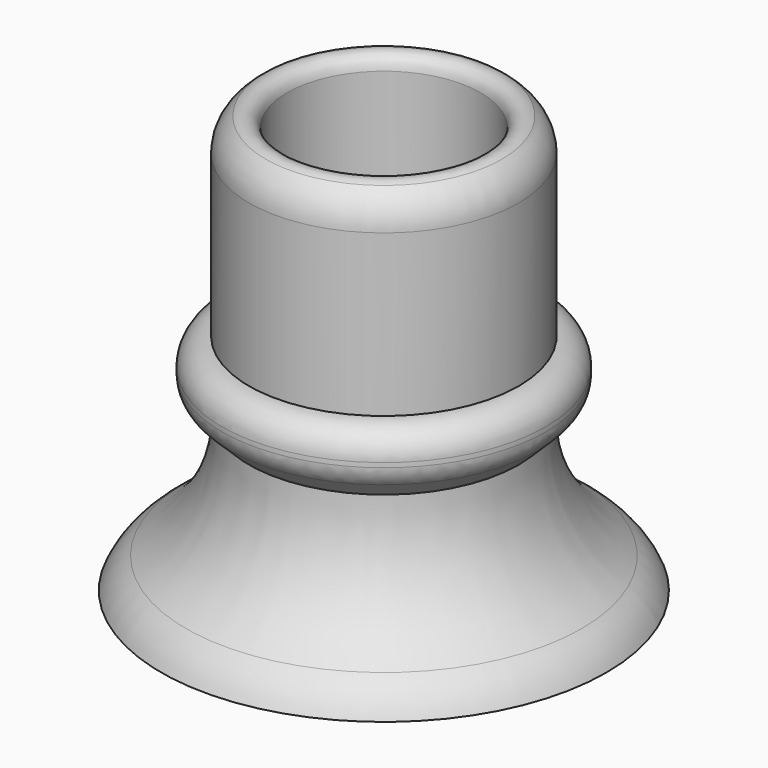
from build123d import *

# Parameters (mm, degrees)
F3_R = 2
F4_R = 2
F6_R = 1


# Not quite as in the source:
# - a fillet or chamfer that OpenCascade refuses, or shapes differently, is made with other operations: its cross-section is extruded or revolved along the edge and cut away or added


with BuildPart() as f1:
    # F0 (on Front) → F1 (revolve)
    with BuildSketch(Plane.XZ):
        with BuildLine():
            ThreePointArc((16.5, 1.2755964417), (11.6628201448, 5.344639677), (10, 11.4430370868))
            Line((10, 11.4430370868), (12, 13.4055894333))
            Line((12, 13.4055894333), (12, 16.5758651609))
            Line((12, 16.5758651609), (9.9997436628, 16.5758651609))
            Line((9.9997436628, 16.5758651609), (9.9997436628, 31.5143950284))
            Line((9.9997436628, 31.5143950284), (7.1613686159, 31.5143950284))
            Line((7.1613686159, 31.5143950284), (7.1613686159, 5.6914240122))
            ThreePointArc((7.1613686159, 5.6914240122), (4.4508587391, 2.967008827), (1, 1.2755964417))
            Line((1, 1.2755964417), (1, 0.0454979338))
            Line((1, 0.0454979338), (16.5, 0))
            Line((16.5, 0), (16.5, 1.2755964417))
        make_face()
    revolve(axis=Axis((0, 0, 19.1986504942), (0, 0, 1)))

    # F2: fillet of radius 5 on 1 edges, made by hand

    # F2_s1 → F2_t2 (revolve, cut)
    with BuildSketch(Plane.XZ):
        with BuildLine():
            ThreePointArc((16.5, 0), (15.750789479, 1.2709297875), (14.6632904097, 2.2678875116))
            ThreePointArc((14.6632904097, 2.2678875116), (15.557168946, 1.7264369439), (16.5, 1.2755964417))
            Line((16.5, 1.2755964417), (16.5, 0))
        make_face()
    revolve(axis=Axis((0, 0, 1.2755964417), (0, 0, 1)), mode=Mode.SUBTRACT)

    # F3
    f3_edges = [f1.edges().sort_by_distance(p)[0] for p in [
        (-12, 0, 13.405589),
    ]]
    fillet(f3_edges, radius=F3_R)

    # F4
    f4_edges = [f1.edges().sort_by_distance(p)[0] for p in [
        (-12, 0, 16.575865),
    ]]
    fillet(f4_edges, radius=F4_R)

    # F5: fillet of radius 3 on 1 edges, made by hand

    # F5_s1 → F5_t2 (revolve, cut)
    with BuildSketch(Plane.XZ):
        with BuildLine():
            ThreePointArc((9.9997436628, 28.5187519631), (9.1774574708, 30.5821381534), (7.1613686159, 31.5143950284))
            Line((7.1613686159, 31.5143950284), (9.9997436628, 31.5143950284))
            Line((9.9997436628, 31.5143950284), (9.9997436628, 28.5187519631))
        make_face()
    revolve(axis=Axis((0, 0, 31.5143950284), (0, 0, 1)), mode=Mode.SUBTRACT)

    # F6
    f6_edges = [f1.edges().sort_by_distance(p)[0] for p in [
        (-7.161369, 0, 31.514395),
    ]]
    fillet(f6_edges, radius=F6_R)


solid = f1.part
